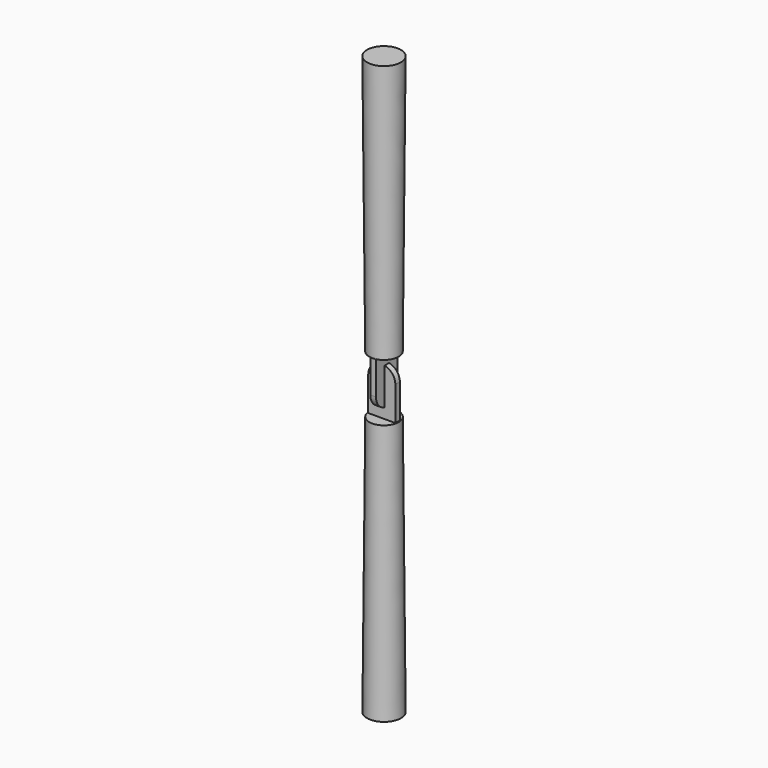
from build123d import *

# Parameters (mm, degrees)
F0_R     = 2
F1_DEPTH = 1.25
F4_W     = 6
F4_H     = 15
F6_DEPTH = 1.25
F7_W     = 6
F7_H     = 15
F9_DEPTH = 1.25


# Not quite as in the source:
# - a feature names something its author has since deleted; it is built from what else it names


with BuildPart() as f1:
    # F0 (on Front) → F1 (new body, symmetric)
    with BuildSketch(Plane.XZ):
        with BuildLine():
            Line((-6, 15), (-6, 0))
            Line((-6, 0), (6, 0))
            Line((6, 0), (6, 6))
            ThreePointArc((6, 6), (4.2426406871, 10.2426406871), (0, 12))
            ThreePointArc((0, 12), (-2.1213203436, 17.1213203436), (3, 15))
            ThreePointArc((3, 15), (4.5, 13.5), (6, 15))
            ThreePointArc((6, 15), (0, 21), (-6, 15))
        make_face()
        with Locations((0, 6)):
            Circle(F0_R, mode=Mode.SUBTRACT)
    extrude(amount=F1_DEPTH, both=True)

    # F2 (on Right) → F3 (revolve)
    with BuildSketch(Plane.YZ):
        Polygon((0, -115), (0, 0), (-6.5, 0), (-7.5, -115), align=None)
    revolve(axis=Axis((0, 0, -57.5), (0, 0, -1)))



with BuildPart() as f5:
    # F4 (on Front) → F5 (revolve)
    with BuildSketch(Plane.XZ):
        Polygon((0, -115), (0, 0), (-6, 0), (-6.5, 0), (-7.5, -115), align=None)
    revolve(axis=Axis((0, 0, -57.5), (0, 0, 1)))


with BuildPart() as f1_1:
    add(f1.part)

    add(f5.part)  # F6 merges F5
    # F4 (on Front) → F6 (join, symmetric)
    with BuildSketch(Plane.XZ):
        with Locations((-3, 7.5)):
            Rectangle(F4_W, F4_H)
        with Locations((3, 7.5)):
            Rectangle(F4_W, F4_H)
        with BuildLine():
            Line((-6, 15), (0, 15))
            Line((0, 15), (6, 15))
            ThreePointArc((6, 15), (0, 21), (-6, 15))
        make_face()
    extrude(amount=F6_DEPTH, both=True)


with BuildPart() as f8:
    # F7 (on Right) → F8 (revolve)
    with BuildSketch(Plane.YZ):
        Polygon((-6, 25.5), (-0.0391304348, 25.5), (-0.0391304348, 140.5), (-7.5391304348, 140.5), (-6.5391304348, 25.5), align=None)
    revolve(axis=Axis((0, -0.0391304348, 83), (0, 0, 1)))


with BuildPart() as f9:
    # F7 (on Right) → F9 (new body, symmetric)
    with BuildSketch(Plane.YZ):
        Polygon((0, 10.5), (0, 25.5), (-0.0391304348, 25.5), (-6, 25.5), (-6, 10.5), align=None)
        with Locations((3, 18)):
            Rectangle(F7_W, F7_H)
        with BuildLine():
            Line((6, 10.5), (0, 10.5))
            Line((0, 10.5), (-6, 10.5))
            ThreePointArc((-6, 10.5), (-4.2426406871, 6.2573593129), (0, 4.5))
            ThreePointArc((0, 4.5), (4.2426406871, 6.2573593129), (6, 10.5))
        make_face()
    extrude(amount=F9_DEPTH, both=True)


solid = Compound([f1_1.part, f8.part, f9.part])
